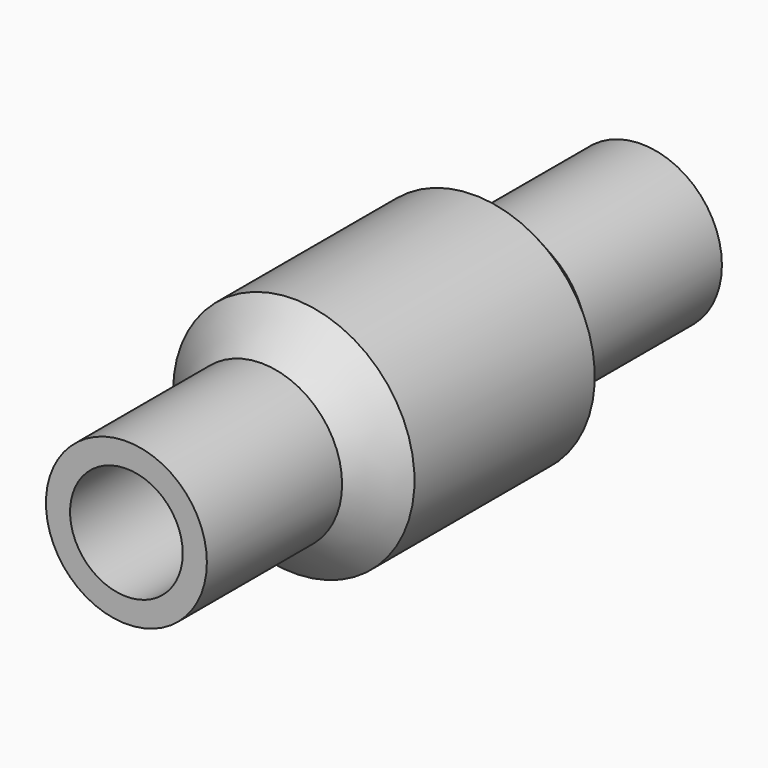
from build123d import *

# Parameters (mm, degrees)
F0_R         = 5
F0_R_2       = 3.5
F1_DEPTH     = 10
F2_R         = 7.5
F2_R_2       = 5
F2_R_3       = 3.5
F3_DEPTH     = 10
F5_S5_R      = 5
F5_T6_DEPTH  = 12
F5_S11_R     = 5
F5_T12_DEPTH = 12


# Not quite as in the source:
# - a fillet or chamfer that OpenCascade refuses, or shapes differently, is made with other operations: its cross-section is extruded or revolved along the edge and cut away or added


with BuildPart() as f1:
    # F0 (on Front) → F1 (new body)
    with BuildSketch(Plane.XZ):
        Circle(F0_R)
        Circle(F0_R_2, mode=Mode.SUBTRACT)
    extrude(amount=F1_DEPTH)

    # F2 (on face) → F3 (join)
    with BuildSketch(Plane(origin=(0, 0, 0), x_dir=(-1, 0, 0), z_dir=(0, 1, 0))):
        Circle(F2_R)
        Circle(F2_R_2, mode=Mode.SUBTRACT)
        Circle(F2_R_2)
        Circle(F2_R_3, mode=Mode.SUBTRACT)
    extrude(amount=F3_DEPTH)

    # F4: F1 across face


with BuildPart() as f1_1:
    add(f1.part)
    add(f1.part.mirror(Plane(origin=(0, 10, 0), x_dir=(-1, 0, 0), z_dir=(0, 1, 0))))

    # F5: chamfer of 3 on 2 edges, made by hand


with BuildPart() as f5_tool2:
    # F5_s3 → F5_t4 (revolve)
    with BuildSketch(Plane.XY):
        Polygon((-4.5, 20), (-7.5, 17), (-7.5, 20), align=None)
    revolve(axis=Axis((0, 20, 0), (0, 1, 0)))

    # F5_s5 → F5_t6 (cut, symmetric)
    with BuildSketch(Plane.XZ.offset(-18.5)):
        Circle(F5_S5_R)
    extrude(amount=F5_T6_DEPTH, both=True, mode=Mode.SUBTRACT)


with BuildPart() as f1_2:
    add(f1_1.part)

    # F5_t1: cut F5_tool2
    add(f5_tool2.part, mode=Mode.SUBTRACT)


with BuildPart() as f5_tool8:
    # F5_s9 → F5_t10 (revolve)
    with BuildSketch(Plane.XY):
        Polygon((-7.5, 3), (-4.5, 0), (-7.5, 0), align=None)
    revolve(axis=Axis((0, 0, 0), (0, 1, 0)))

    # F5_s11 → F5_t12 (cut, symmetric)
    with BuildSketch(Plane.XZ.offset(-1.5)):
        Circle(F5_S11_R)
    extrude(amount=F5_T12_DEPTH, both=True, mode=Mode.SUBTRACT)


with BuildPart() as f1_3:
    add(f1_2.part)

    # F5_t7: cut F5_tool8
    add(f5_tool8.part, mode=Mode.SUBTRACT)


solid = f1_3.part
